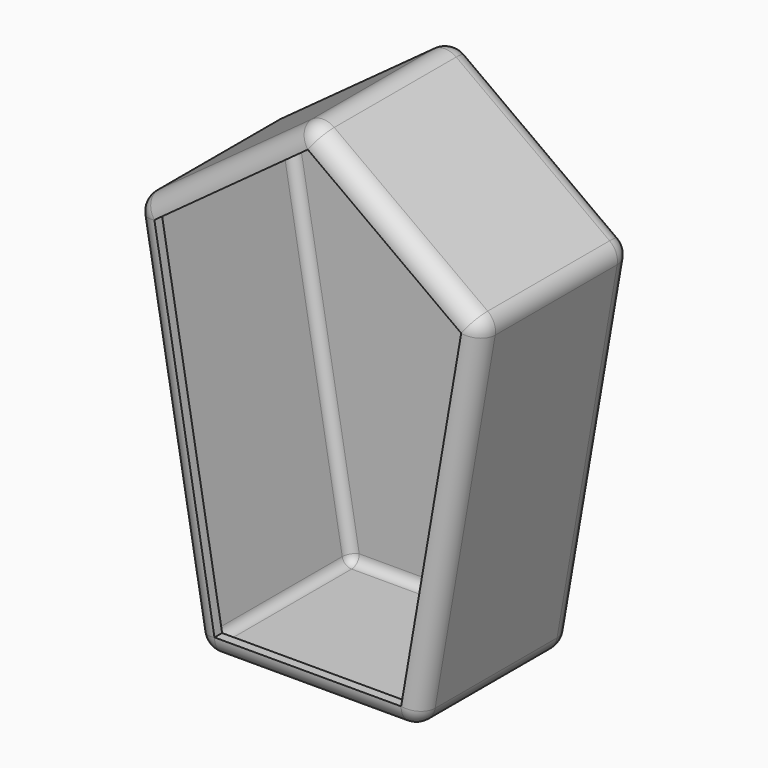
from build123d import *

# Parameters (mm, degrees)
F1_DEPTH = 50.8
F2_R     = 5.08
F3_T     = -2.54


# Not quite as in the source:
# - a shell that OpenCascade refuses in one call is made with other operations: the cavity is built on its own and cut out


with BuildPart() as f1:
    # F0 (on Front) → F1 (new body)
    with BuildSketch(Plane.XZ):
        Polygon((-46.4516356587, 59.1254718602), (-29.1618652595, -40.9925776591), (-21.6381347405, -40.9925776591), (21.6381347405, -40.9925776591), (29.1618652595, -40.9925776591), (46.4516356587, 59.1254718602), (0, 92.9853990674), align=None)
    extrude(amount=F1_DEPTH)

    # F2
    f2_edges = [f1.edges().sort_by_distance(p)[0] for p in [
        (23.225818, -50.8, 76.055435),
        (-23.225818, -50.8, 76.055435),
        (-37.80675, -50.8, 9.066447),
        (0, -50.8, -40.992578),
        (37.80675, -50.8, 9.066447),
        (29.161865, -25.4, -40.992578),
        (46.451636, -25.4, 59.125472),
        (37.80675, 0, 9.066447),
        (23.225818, 0, 76.055435),
        (-23.225818, 0, 76.055435),
        (-37.80675, 0, 9.066447),
        (0, 0, -40.992578),
        (-46.451636, -25.4, 59.125472),
        (-29.161865, -25.4, -40.992578),
        (0, -25.4, 92.985399),
    ]]
    fillet(f2_edges, radius=F2_R)

    # F3: a shell. OpenCascade refuses it in one call, so the cavity is built on its own and cut out:
    # the body offset inwards by the wall thickness, plus a prism from it out through each open face.
    f3_core = offset(f1.part, amount=F3_T, mode=Mode.PRIVATE)
    f3_exits = [f3_core.faces().sort_by_distance(p)[0] for p in [
        (0, -48.26, 23.00503),
    ]]
    add(f3_core, mode=Mode.SUBTRACT)
    extrude(f3_exits, amount=-F3_T, mode=Mode.SUBTRACT)


solid = f1.part
